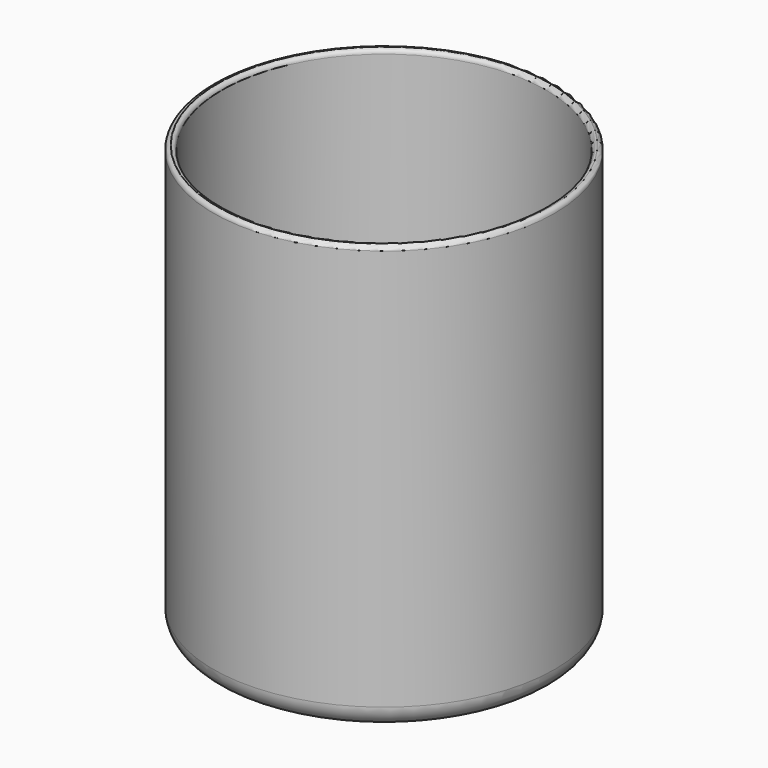
from build123d import *

# Parameters (mm, degrees)
F0_R     = 40
F1_DEPTH = 100
F2_T     = -2
F3_R     = 1
F4_R     = 0.99999
F5_R     = 5


# Not quite as in the source:
# - a fillet or chamfer is up to 0.001 mm smaller than in the source, because OpenCascade refuses the exact size


with BuildPart() as f1:
    # F0 (on Top) → F1 (new body)
    with BuildSketch(Plane.XY):
        Circle(F0_R)
    extrude(amount=F1_DEPTH)

    # F2
    f2_openings = [f1.faces().sort_by_distance(p)[0] for p in [
        (0, 0, 100),
    ]]
    offset(amount=F2_T, openings=f2_openings)

    # F3
    f3_edges = [f1.edges().sort_by_distance(p)[0] for p in [
        (-38, 0, 100),
    ]]
    fillet(f3_edges, radius=F3_R)

    # F4 (radius 1 in the source; OpenCascade refuses exactly that, so slightly less here)
    f4_edges = [f1.edges().sort_by_distance(p)[0] for p in [
        (-40, 0, 100),
    ]]
    fillet(f4_edges, radius=F4_R)

    # F5
    f5_edges = [f1.edges().sort_by_distance(p)[0] for p in [
        (-40, 0, 0),
    ]]
    fillet(f5_edges, radius=F5_R)


solid = f1.part
